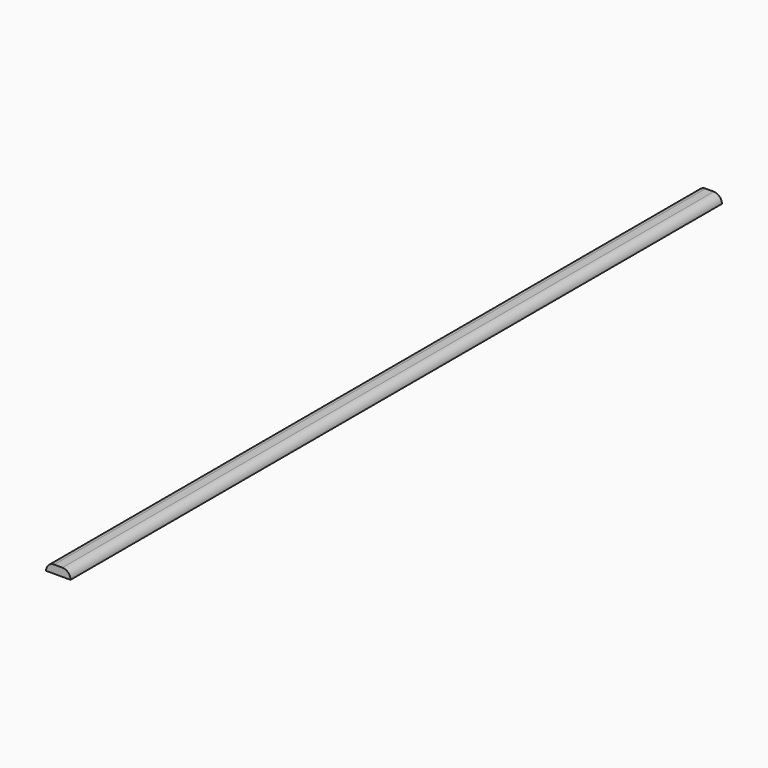
from build123d import *

# Parameters (mm, degrees)
F0_W     = 9.525
F0_H     = 3.175
F1_DEPTH = 317.5
F2_R     = 3.17499


# Not quite as in the source:
# - a fillet or chamfer is up to 0.001 mm smaller than in the source, because OpenCascade refuses the exact size


with BuildPart() as f1:
    # F0 (on Front) → F1 (new body)
    with BuildSketch(Plane.XZ):
        Rectangle(F0_W, F0_H)
    extrude(amount=F1_DEPTH)

    # F2 (radius 3.175 in the source; OpenCascade refuses exactly that, so slightly less here)
    f2_edges = [f1.edges().sort_by_distance(p)[0] for p in [
        (-4.7625, -158.75, 1.5875),
        (4.7625, -158.75, 1.5875),
    ]]
    fillet(f2_edges, radius=F2_R)


solid = f1.part
